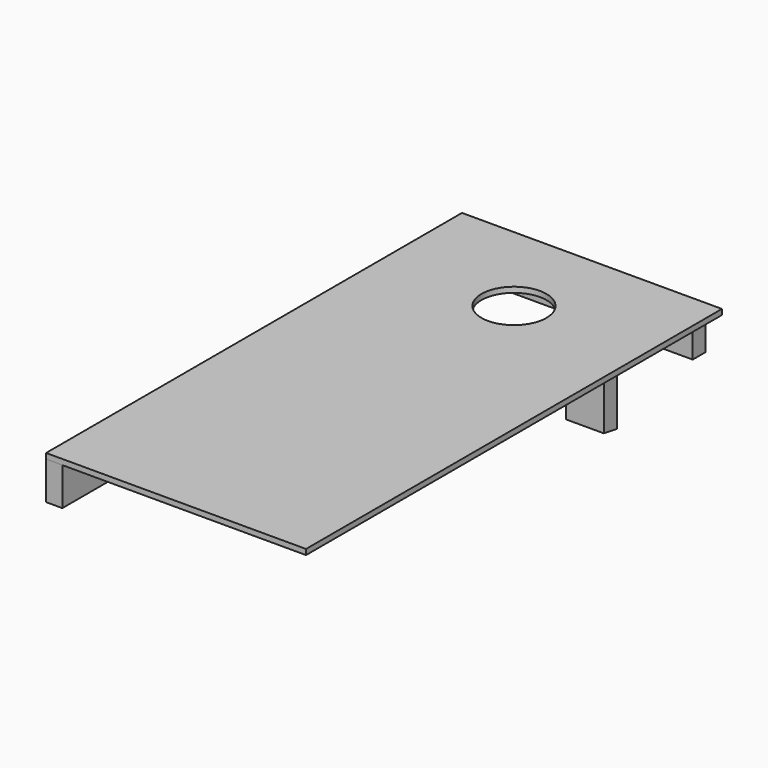
from build123d import *

# Parameters (mm, degrees)
F2_R     = 76.2
F2_W     = 88.9
F2_H     = 38.1
F2_W_2   = 533.4
F2_H_2   = 552.45
F3_DEPTH = 12.7
F4_DEPTH = 88.9
F5_DEPTH = 88.9
F7_DEPTH = 88.9
F8_R     = 3.175
F9_DEPTH = 12.7


with BuildPart() as f3:
    # F2 (on Top) → F3 (new body)
    with BuildSketch(Plane.XY):
        Polygon((266.7, 19.05), (266.7, 571.5), (241.3, 571.5), (241.3, 533.4), (152.4, 533.4), (152.4, 571.5), (-152.4, 571.5), (-152.4, 533.4), (-241.3, 533.4), (-241.3, 571.5), (-266.7, 571.5), (-266.7, 19.05), align=None)
        with Locations((0, 381)):
            Circle(F2_R, mode=Mode.SUBTRACT)
        with Locations((-196.85, 552.45)):
            Rectangle(F2_W, F2_H)
        with Locations((196.85, 552.45)):
            Rectangle(F2_W, F2_H)
        Polygon((266.7, -609.6), (304.8, -609.6), (304.8, 609.6), (266.7, 609.6), (266.7, 571.5), (266.7, 19.05), (266.7, -19.05), (266.7, -571.5), align=None)
        Polygon((-304.8, -609.6), (-266.7, -609.6), (-266.7, -571.5), (-266.7, -19.05), (-266.7, 19.05), (-266.7, 571.5), (-266.7, 609.6), (-304.8, 609.6), align=None)
        Polygon((266.7, 571.5), (266.7, 609.6), (-266.7, 609.6), (-266.7, 571.5), (-241.3, 571.5), (-152.4, 571.5), (152.4, 571.5), (241.3, 571.5), align=None)
        with Locations((0, -590.55)):
            Rectangle(F2_W_2, F2_H)
        with Locations((0, -295.275)):
            Rectangle(F2_W_2, F2_H_2)
        Rectangle(F2_W_2, F2_H)
    extrude(amount=F3_DEPTH)


with BuildPart() as f4:
    # F2 (on Top) → F4 (new body)
    with BuildSketch(Plane.XY):
        Polygon((266.7, 571.5), (266.7, 609.6), (-266.7, 609.6), (-266.7, 571.5), (-241.3, 571.5), (-152.4, 571.5), (152.4, 571.5), (241.3, 571.5), align=None)
    extrude(amount=-F4_DEPTH)

    # F8 (on face) → F9 (cut)
    with BuildSketch(Plane(origin=(0, 609.6, 0), x_dir=(-1, 0, 0), z_dir=(0, 1, 0))):
        with Locations((-254, -63.5)):
            Circle(F8_R)
        with Locations((-254, -25.4)):
            Circle(F8_R)
        with Locations((-228.6, -63.5)):
            Circle(F8_R)
        with Locations((-228.6, -25.4)):
            Circle(F8_R)
        with Locations((-203.2, -63.5)):
            Circle(F8_R)
        with Locations((-203.2, -25.4)):
            Circle(F8_R)
        with Locations((-177.8, -63.5)):
            Circle(F8_R)
        with Locations((-177.8, -25.4)):
            Circle(F8_R)
        with Locations((-152.4, -63.5)):
            Circle(F8_R)
        with Locations((-152.4, -25.4)):
            Circle(F8_R)
        with Locations((-127, -63.5)):
            Circle(F8_R)
        with Locations((-127, -25.4)):
            Circle(F8_R)
        with Locations((-101.6, -63.5)):
            Circle(F8_R)
        with Locations((-101.6, -25.4)):
            Circle(F8_R)
        with Locations((-76.2, -63.5)):
            Circle(F8_R)
        with Locations((-76.2, -25.4)):
            Circle(F8_R)
        with Locations((-50.8, -63.5)):
            Circle(F8_R)
        with Locations((-50.8, -25.4)):
            Circle(F8_R)
        with Locations((-25.4, -63.5)):
            Circle(F8_R)
        with Locations((-25.4, -25.4)):
            Circle(F8_R)
        with Locations((0, -63.5)):
            Circle(F8_R)
        with Locations((0, -25.4)):
            Circle(F8_R)
        with Locations((25.4, -63.5)):
            Circle(F8_R)
        with Locations((25.4, -25.4)):
            Circle(F8_R)
        with Locations((50.8, -63.5)):
            Circle(F8_R)
        with Locations((50.8, -25.4)):
            Circle(F8_R)
        with Locations((76.2, -63.5)):
            Circle(F8_R)
        with Locations((76.2, -25.4)):
            Circle(F8_R)
        with Locations((101.6, -63.5)):
            Circle(F8_R)
        with Locations((101.6, -25.4)):
            Circle(F8_R)
        with Locations((127, -63.5)):
            Circle(F8_R)
        with Locations((127, -25.4)):
            Circle(F8_R)
        with Locations((152.4, -63.5)):
            Circle(F8_R)
        with Locations((152.4, -25.4)):
            Circle(F8_R)
        with Locations((177.8, -63.5)):
            Circle(F8_R)
        with Locations((177.8, -25.4)):
            Circle(F8_R)
        with Locations((203.2, -63.5)):
            Circle(F8_R)
        with Locations((203.2, -25.4)):
            Circle(F8_R)
        with Locations((228.6, -63.5)):
            Circle(F8_R)
        with Locations((228.6, -25.4)):
            Circle(F8_R)
        with Locations((254, -63.5)):
            Circle(F8_R)
        with Locations((254, -25.4)):
            Circle(F8_R)
    extrude(amount=-F9_DEPTH, mode=Mode.SUBTRACT)


with BuildPart() as f5:
    # F2 (on Top) → F5 (new body)
    with BuildSketch(Plane.XY):
        Polygon((-304.8, -609.6), (-266.7, -609.6), (-266.7, -571.5), (-266.7, -19.05), (-266.7, 19.05), (-266.7, 571.5), (-266.7, 609.6), (-304.8, 609.6), align=None)
    extrude(amount=-F5_DEPTH)


with BuildPart() as f7:
    # F6 (on Right) → F7 (new body)
    with BuildSketch(Plane.YZ):
        Polygon((571.5, -289.9994348001), (571.5, 0), (533.4, 0), (533.4, -283.5123562581), align=None)
    extrude(amount=F7_DEPTH)


solid = Compound([f3.part, f4.part, f5.part, f7.part])
